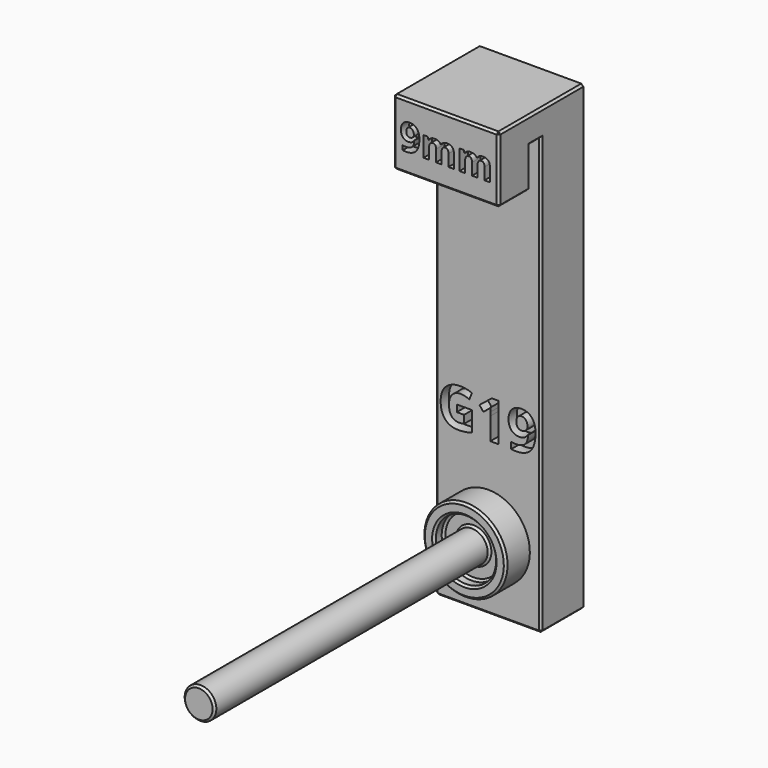
from build123d import *

# Parameters (mm, degrees)
F1_DEPTH     = 12.7
F4_SIZE      = 0.5
F5_TEXT_SIZE = 8.8194444444
F6_DEPTH     = 2.5
F7_SIZE      = 0.5
F8_TEXT_SIZE = 12.8706832605
F9_DEPTH     = 2.5


# Not quite as in the source:
# - Text() gives the source's letters only with a copy of the font that has no kerning and outlines rounded to 1/6400 em; it was checked with that copy


with BuildPart() as f1:
    # F0 (on Right) → F1 (new body, symmetric)
    with BuildSketch(Plane.YZ):
        Polygon((12.7, 55.5625), (-12.7, 55.5625), (-12.7, 39.6875), (-3.302, 39.6875), (-3.302, 49.2125), (0, 49.2125), (0, -55.5625), (12.7, -55.5625), align=None)
    extrude(amount=F1_DEPTH, both=True)

    # F2 (on Right) → F3 (revolve)
    with BuildSketch(Plane.YZ):
        Polygon((-86.995, -39.2125), (0, -39.2125), (0, -31.9625), (0, -29.2125), (-7.195, -29.2125), (-7.195, -31.9625), (-4.445, -31.9625), (-4.445, -35.4025), (-86.995, -35.4025), align=None)
    revolve(axis=Axis((0, 0, -39.2125), (0, 1, 0)))

    # F4
    f4_edges = [f1.edges().sort_by_distance(p)[0] for p in [
        (-12.7, 0, 55.5625),
        (-12.7, 0, -3.175),
        (-12.7, 6.35, -55.5625),
        (-12.7, -1.651, 49.2125),
        (-12.7, -3.302, 44.45),
        (-12.7, -12.7, 47.625),
        (-12.7, -8.001, 39.6875),
        (12.7, 6.35, -55.5625),
        (12.7, 0, 55.5625),
        (12.7, -12.7, 47.625),
        (12.7, -1.651, 49.2125),
        (12.7, -3.302, 44.45),
        (12.7, -8.001, 39.6875),
        (12.7, 0, -3.175),
        (0, 0, -55.5625),
        (0, -12.7, 55.5625),
        (0, -12.7, 39.6875),
        (0, -3.302, 39.6875),
        (0, -86.995, -43.0225),
        (0, -4.445, -46.4625),
    ]]
    chamfer(f4_edges, length=F4_SIZE)

    # F5 (on face) → F6 (cut)
    with BuildSketch(Plane.XZ.offset(12.7)):
        with Locations((-11.1331705729, 44.45)):
            Text('9mm', F5_TEXT_SIZE, font='Open Sans', font_style=FontStyle.BOLD, text_align=(TextAlign.LEFT, TextAlign.BOTTOM))
    extrude(amount=-F6_DEPTH, mode=Mode.SUBTRACT)

    # F7
    f7_edges = [f1.edges().sort_by_distance(p)[0] for p in [
        (0, -7.195, -46.4625),
        (0, -7.195, -49.2125),
        (0, -4.445, -43.0225),
    ]]
    chamfer(f7_edges, length=F7_SIZE)

    # F8 (on face) → F9 (cut)
    with BuildSketch(Plane.XZ):
        with Locations((-12.2, -18.7918919476)):
            Text('G19', F8_TEXT_SIZE, font='Open Sans', font_style=FontStyle.BOLD, text_align=(TextAlign.LEFT, TextAlign.BOTTOM))
    extrude(amount=-F9_DEPTH, mode=Mode.SUBTRACT)


solid = f1.part
